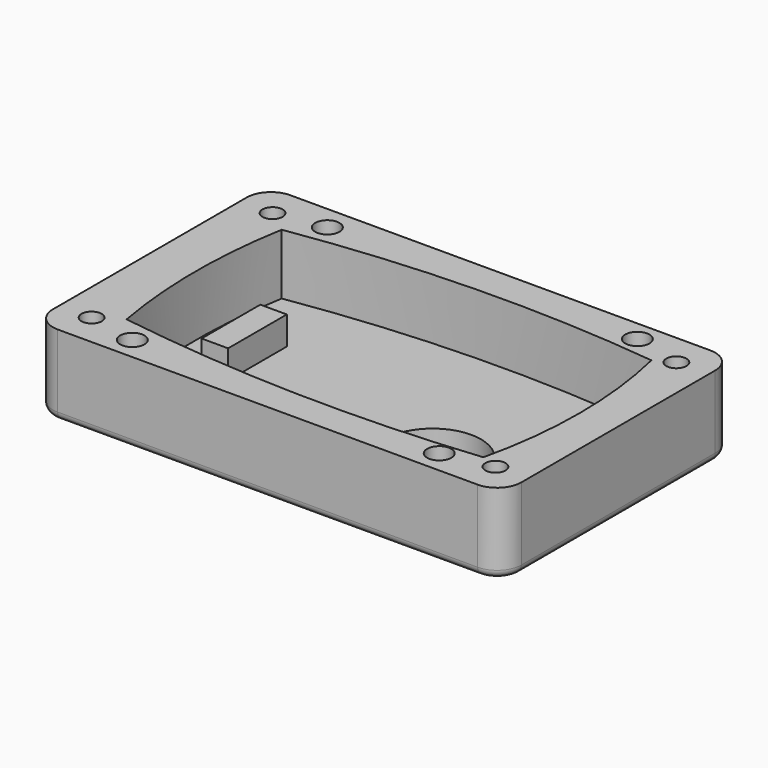
from build123d import *

# Parameters (mm, degrees)
F0_W     = 58
F0_H     = 36
F0_R     = 1.25
F0_R_2   = 1.5
F1_DEPTH = 10
F0_R_3   = 1
F0_W_2   = 3.2825097442
F0_H_2   = 9.0816104785
F2_DEPTH = 2.5
F3_R     = 3
F4_DEPTH = 6
F5_START = 0.9
F5_DEPTH = 16.2
F6_START = 6
F6_DEPTH = 10.7
F7_R     = 1


with BuildPart() as f1:
    # F0 (on Top) → F1 (new body)
    with BuildSketch(Plane.XY):
        with Locations((22.1260370687, 12.181818096)):
            Rectangle(F0_W, F0_H)
        with Locations((-2.8739629313, -1.818181904)):
            Circle(F0_R, mode=Mode.SUBTRACT)
        with Locations((3.1260370687, -3.018181904)):
            Circle(F0_R_2, mode=Mode.SUBTRACT)
        with Locations((41.1260370687, -3.018181904)):
            Circle(F0_R_2, mode=Mode.SUBTRACT)
        with Locations((47.1260370687, -1.818181904)):
            Circle(F0_R, mode=Mode.SUBTRACT)
        with BuildLine():
            Line((-0.0042433119, 0.0237876128), (-0.0123524841, 0.02397218))
            Line((-0.0123524841, 0.02397218), (-0.0123524841, 0.0693824727))
            ThreePointArc((-0.0123524841, 0.0693824727), (-1.0671188126, 12.0466773263), (-0.0123524841, 24.02397218))
            ThreePointArc((-0.0123524841, 24.02397218), (22.4498159336, 26.0118318189), (44.9770614896, 25))
            ThreePointArc((44.9770614896, 25), (46.474513746, 12), (44.9770614896, -1))
            ThreePointArc((44.9770614896, -1), (22.4574664967, -1.8971785964), (0, 0))
            ThreePointArc((0, 0), (-0.0021227043, 0.0118936194), (-0.0042433119, 0.0237876128))
        make_face(mode=Mode.SUBTRACT)
        with Locations((-2.8739629313, 26.181818096)):
            Circle(F0_R, mode=Mode.SUBTRACT)
        with Locations((3.1260370687, 27.16396598)):
            Circle(F0_R_2, mode=Mode.SUBTRACT)
        with Locations((41.1260370687, 27.6376707083)):
            Circle(F0_R_2, mode=Mode.SUBTRACT)
        with Locations((47.1260370687, 26.181818096)):
            Circle(F0_R, mode=Mode.SUBTRACT)
        with Locations((-2.8739629313, 26.181818096)):
            Circle(F0_R)
        with Locations((47.1260370687, 26.181818096)):
            Circle(F0_R)
        with Locations((47.1260370687, -1.818181904)):
            Circle(F0_R)
        with Locations((-2.8739629313, -1.818181904)):
            Circle(F0_R)
        with Locations((3.1260370687, -3.018181904)):
            Circle(F0_R_2)
        with Locations((3.1260370687, 27.16396598)):
            Circle(F0_R_2)
        with Locations((41.1260370687, 27.6376707083)):
            Circle(F0_R_2)
        with Locations((41.1260370687, -3.018181904)):
            Circle(F0_R_2)
    extrude(amount=F1_DEPTH)

    # F0 (on Top) → F2 (join)
    with BuildSketch(Plane.XY):
        with BuildLine():
            ThreePointArc((-0.0123524841, 24.02397218), (-1.0671188126, 12.0466773263), (-0.0123524841, 0.0693824727))
            Line((-0.0123524841, 0.0693824727), (-0.0123524841, 24.02397218))
        make_face()
        with BuildLine():
            Line((-0.0123524841, 24.02397218), (-0.0123524841, 0.0693824727))
            ThreePointArc((-0.0123524841, 0.0693824727), (-0.0083017494, 0.0465843578), (-0.0042433119, 0.0237876128))
            Line((-0.0042433119, 0.0237876128), (44.9770614896, -1))
            Line((44.9770614896, -1), (44.9770614896, 25))
            Line((44.9770614896, 25), (-0.0123524841, 24.02397218))
        make_face()
        with Locations((2.9621722015, 2.0848012064)):
            Circle(F0_R_3, mode=Mode.SUBTRACT)
        with Locations((5.0146379508, 11.9371688925)):
            Rectangle(F0_W_2, F0_H_2, mode=Mode.SUBTRACT)
        with Locations((41.7125664489, 2.0848012064)):
            Circle(F0_R_3, mode=Mode.SUBTRACT)
        with BuildLine():
            Line((26.1260370687, 7.1930042468), (26.1260370687, 9.181818096))
            Line((26.1260370687, 9.181818096), (26.4652403515, 9.181818096))
            ThreePointArc((26.4652403515, 9.181818096), (32.1260370687, 13.1930042468), (37.7868337859, 9.181818096))
            Line((37.7868337859, 9.181818096), (38.1260370687, 9.181818096))
            Line((38.1260370687, 9.181818096), (38.1260370687, 7.1930042468))
            Line((38.1260370687, 7.1930042468), (38.1260370687, 1.181818096))
            Line((38.1260370687, 1.181818096), (26.1260370687, 1.181818096))
            Line((26.1260370687, 1.181818096), (26.1260370687, 7.1930042468))
        make_face(mode=Mode.SUBTRACT)
        with Locations((41.1260370687, 12.181818096)):
            Circle(F0_R_2, mode=Mode.SUBTRACT)
        with Locations((18.8074270263, 12.2937392443)):
            Circle(F0_R_3, mode=Mode.SUBTRACT)
        with Locations((2.9621722015, 21.6664075851)):
            Circle(F0_R_3, mode=Mode.SUBTRACT)
        with Locations((26.8074270263, 12.2937392443)):
            Circle(F0_R_3, mode=Mode.SUBTRACT)
        with Locations((41.7125664489, 21.6664075851)):
            Circle(F0_R_3, mode=Mode.SUBTRACT)
        with BuildLine():
            Line((44.9770614896, -1), (-0.0042433119, 0.0237876128))
            ThreePointArc((-0.0042433119, 0.0237876128), (-0.0021227043, 0.0118936194), (0, 0))
            ThreePointArc((0, 0), (22.4574664967, -1.8971785964), (44.9770614896, -1))
        make_face()
        with BuildLine():
            ThreePointArc((44.9770614896, 25), (22.4498159336, 26.0118318189), (-0.0123524841, 24.02397218))
            Line((-0.0123524841, 24.02397218), (44.9770614896, 25))
        make_face()
        with BuildLine():
            Line((44.9770614896, 25), (44.9770614896, -1))
            ThreePointArc((44.9770614896, -1), (46.474513746, 12), (44.9770614896, 25))
        make_face()
        with Locations((2.9621722015, 21.6664075851)):
            Circle(F0_R_3)
        with Locations((2.9621722015, 2.0848012064)):
            Circle(F0_R_3)
        with Locations((41.7125664489, 2.0848012064)):
            Circle(F0_R_3)
        with Locations((41.7125664489, 21.6664075851)):
            Circle(F0_R_3)
        with Locations((18.8074270263, 12.2937392443)):
            Circle(F0_R_3)
        with Locations((26.8074270263, 12.2937392443)):
            Circle(F0_R_3)
        with Locations((5.0146379508, 11.9371688925)):
            Rectangle(F0_W_2, F0_H_2)
        with BuildLine():
            Line((26.4652403515, 9.181818096), (26.1260370687, 9.181818096))
            Line((26.1260370687, 9.181818096), (26.1260370687, 7.1930042468))
            ThreePointArc((26.1260370687, 7.1930042468), (26.2114457767, 8.2017707453), (26.4652403515, 9.181818096))
        make_face()
        with BuildLine():
            ThreePointArc((38.1260370687, 7.1930042468), (32.1260370687, 1.1930042468), (26.1260370687, 7.1930042468))
            Line((26.1260370687, 7.1930042468), (26.1260370687, 1.181818096))
            Line((26.1260370687, 1.181818096), (38.1260370687, 1.181818096))
            Line((38.1260370687, 1.181818096), (38.1260370687, 7.1930042468))
        make_face()
        with BuildLine():
            Line((38.1260370687, 9.181818096), (37.7868337859, 9.181818096))
            ThreePointArc((37.7868337859, 9.181818096), (38.0406283607, 8.2017707453), (38.1260370687, 7.1930042468))
            Line((38.1260370687, 7.1930042468), (38.1260370687, 9.181818096))
        make_face()
    extrude(amount=F2_DEPTH)

    # F3
    f3_edges = [f1.edges().sort_by_distance(p)[0] for p in [
        (51.126037, 30.181818, 5),
        (51.126037, -5.818182, 5),
        (-6.873963, -5.818182, 5),
        (-6.873963, 30.181818, 5),
    ]]
    fillet(f3_edges, radius=F3_R)

    # F0 (on Top) → F4 (join)
    with BuildSketch(Plane.XY):
        with Locations((5.0146379508, 11.9371688925)):
            Rectangle(F0_W_2, F0_H_2)
    extrude(amount=F4_DEPTH)

    # F0 (on Top) → F5 (cut)
    with BuildSketch(Plane.XY.offset(F5_START)):
        with Locations((47.1260370687, 26.181818096)):
            Circle(F0_R)
        with Locations((-2.8739629313, 26.181818096)):
            Circle(F0_R)
        with Locations((-2.8739629313, -1.818181904)):
            Circle(F0_R)
        with Locations((47.1260370687, -1.818181904)):
            Circle(F0_R)
    extrude(amount=F5_DEPTH, mode=Mode.SUBTRACT)

    # F0 (on Top) → F6 (cut)
    with BuildSketch(Plane.XY.offset(F6_START)):
        with Locations((3.1260370687, 27.16396598)):
            Circle(F0_R_2)
        with Locations((41.1260370687, 27.6376707083)):
            Circle(F0_R_2)
        with Locations((41.1260370687, -3.018181904)):
            Circle(F0_R_2)
        with Locations((3.1260370687, -3.018181904)):
            Circle(F0_R_2)
    extrude(amount=F6_DEPTH, mode=Mode.SUBTRACT)

    # F7
    f7_edges = [f1.edges().sort_by_distance(p)[0] for p in [
        (51.126037, 12.181818, 0),
        (22.126037, -5.818182, 0),
        (50.247357, -4.939502, 0),
        (50.247357, 29.303138, 0),
        (22.126037, 30.181818, 0),
        (-5.995283, 29.303138, 0),
        (-6.873963, 12.181818, 0),
        (-5.995283, -4.939502, 0),
    ]]
    fillet(f7_edges, radius=F7_R)


solid = f1.part
